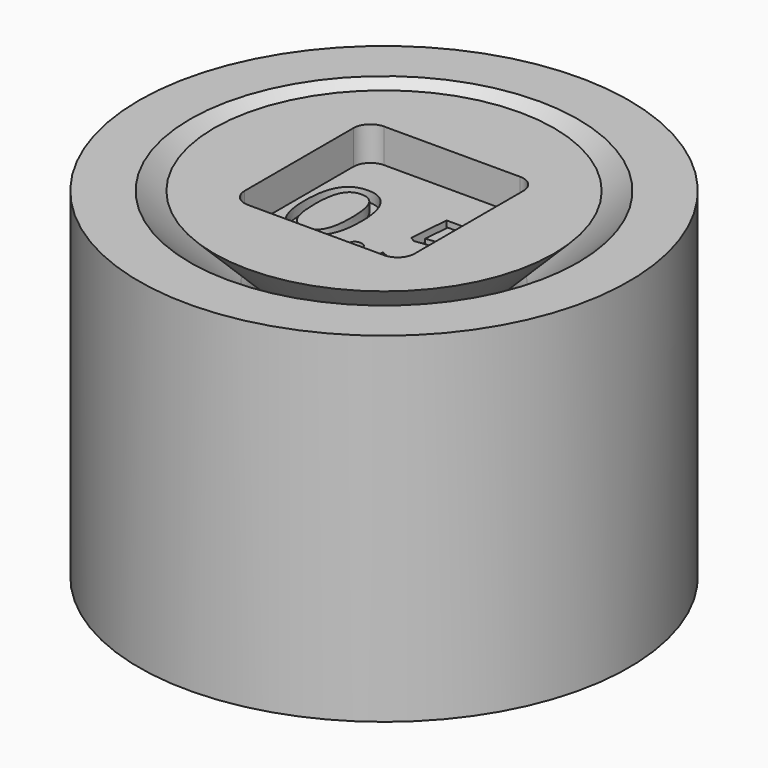
from build123d import *

# Parameters (mm, degrees)
F4_DEPTH     = 1
F5_TEXT_SIZE = 3.5288928099
F6_DEPTH     = 1.3


# Not quite as in the source:
# - Text() gives the source's letters only with a copy of the font that has no kerning and outlines rounded to 1/6400 em; it was checked with that copy


with BuildPart() as f1:
    # F0 (on Front) → F1 (revolve)
    with BuildSketch(Plane.XZ):
        with BuildLine():
            Line((-5, 0), (0, 0))
            Line((0, 0), (0, 10))
            Line((0, 10), (-5, 10))
            Line((-5, 10), (-2.7928932188, 7.7928932188))
            ThreePointArc((-2.7928932188, 7.7928932188), (-2.5761204675, 7.46846987), (-2.5, 7.0857864376))
            Line((-2.5, 7.0857864376), (-2.5, 2.9142135624))
            ThreePointArc((-2.5, 2.9142135624), (-2.5761204675, 2.53153013), (-2.7928932188, 2.2071067812))
            Line((-2.7928932188, 2.2071067812), (-5, 0))
        make_face()
    revolve(axis=Axis((0, 0, 5), (0, 0, 1)))

    # F3 (on face) → F4 (cut)
    with BuildSketch(Plane.XY.offset(10)):
        with BuildLine():
            Line((2, 2.5), (-2, 2.5))
            ThreePointArc((-2, 2.5), (-2.3535533906, 2.3535533906), (-2.5, 2))
            Line((-2.5, 2), (-2.5, -2))
            ThreePointArc((-2.5, -2), (-2.3535533906, -2.3535533906), (-2, -2.5))
            Line((-2, -2.5), (2, -2.5))
            ThreePointArc((2, -2.5), (2.3535533906, -2.3535533906), (2.5, -2))
            Line((2.5, -2), (2.5, 2))
            ThreePointArc((2.5, 2), (2.3535533906, 2.3535533906), (2, 2.5))
        make_face()
    extrude(amount=-F4_DEPTH, mode=Mode.SUBTRACT)

    # F5 (on offset) → F6 (cut)
    with BuildSketch(Plane.XY.offset(10)):
        with Locations((-2.5, -1.2704014116)):
            Text('0.5', F5_TEXT_SIZE, font='Open Sans', text_align=(TextAlign.LEFT, TextAlign.BOTTOM))
    extrude(amount=-F6_DEPTH, mode=Mode.SUBTRACT)


with BuildPart() as f1b:
    # F0 (on Front) → F1, piece 2 (revolve)
    with BuildSketch(Plane.XZ):
        with BuildLine():
            Line((-7.2071067812, 10), (-7.2071067812, 0))
            Line((-7.2071067812, 0), (-5.7071067812, 0))
            Line((-5.7071067812, 0), (-3.2928932188, 2.4142135624))
            ThreePointArc((-3.2928932188, 2.4142135624), (-3.0761204675, 2.7386369112), (-3, 3.1213203436))
            Line((-3, 3.1213203436), (-3, 6.8786796564))
            ThreePointArc((-3, 6.8786796564), (-3.0761204675, 7.2613630888), (-3.2928932188, 7.5857864376))
            Line((-3.2928932188, 7.5857864376), (-5.7071067812, 10))
            Line((-5.7071067812, 10), (-7.2071067812, 10))
        make_face()
    revolve(axis=Axis((0, 0, 5), (0, 0, 1)))


solid = Compound([f1.part, f1b.part])
